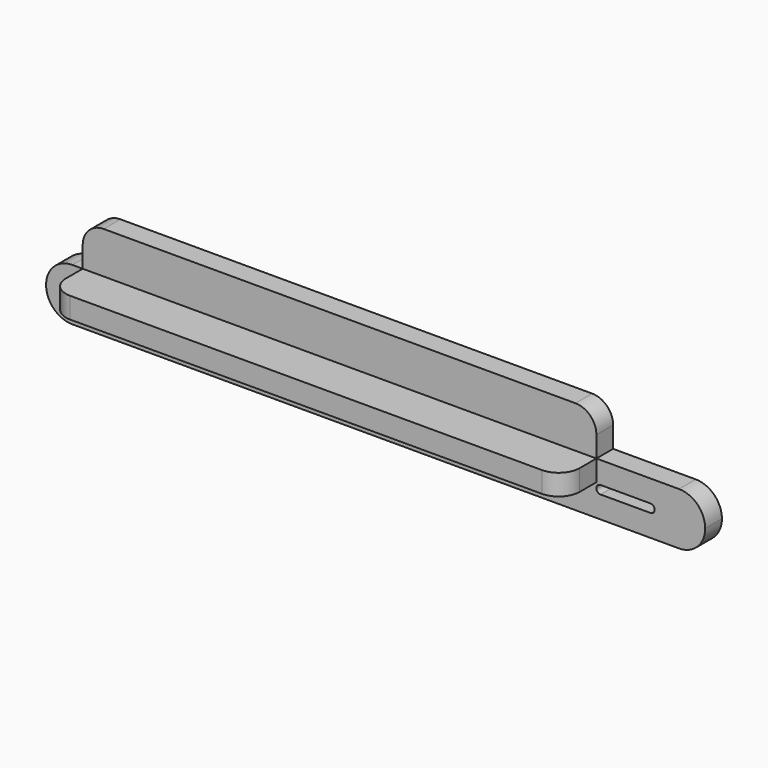
from build123d import *

# Parameters (mm, degrees)
F0_W     = 315
F0_H     = 25
F0_R     = 2.5
F1_DEPTH = 10
F2_R     = 12.49999
F3_W     = 245.5
F3_H     = 10
F4_DEPTH = 20
F5_W     = 245.5
F5_H     = 10
F6_DEPTH = 20
F7_R     = 10
F8_R     = 10


# Not quite as in the source:
# - a fillet or chamfer is up to 0.001 mm smaller than in the source, because OpenCascade refuses the exact size


with BuildPart() as f1:
    # F0 (on Front) → F1 (new body)
    with BuildSketch(Plane.XZ):
        with Locations((167.5, 12.5)):
            Rectangle(F0_W, F0_H)
        with Locations((25, 12.5)):
            Circle(F0_R, mode=Mode.SUBTRACT)
        with BuildLine():
            ThreePointArc((298.861, 14.5), (300.861, 12.5), (298.861, 10.5))
            Line((298.861, 10.5), (275, 10.5))
            ThreePointArc((275, 10.5), (273, 12.5), (275, 14.5))
            Line((275, 14.5), (298.861, 14.5))
        make_face(mode=Mode.SUBTRACT)
    extrude(amount=F1_DEPTH)

    # F2 (radius 12.5 in the source; OpenCascade refuses exactly that, so slightly less here)
    f2_edges = [f1.edges().sort_by_distance(p)[0] for p in [
        (10, -5, 25),
        (10, -5, 0),
        (325, -5, 0),
        (325, -5, 25),
    ]]
    fillet(f2_edges, radius=F2_R)

    # F3 (on face) → F4 (join)
    with BuildSketch(Plane.XZ.offset(10)):
        with Locations((150.25, 20)):
            Rectangle(F3_W, F3_H)
    extrude(amount=F4_DEPTH)

    # F5 (on face) → F6 (join)
    with BuildSketch(Plane.XY.offset(25)):
        with Locations((150.25, -5)):
            Rectangle(F5_W, F5_H)
    extrude(amount=F6_DEPTH)

    # F7
    f7_edges = [f1.edges().sort_by_distance(p)[0] for p in [
        (27.5, -5, 45),
    ]]
    fillet(f7_edges, radius=F7_R)

    # F8
    f8_edges = [f1.edges().sort_by_distance(p)[0] for p in [
        (273, -5, 45),
        (273, -30, 20),
        (27.5, -30, 20),
    ]]
    fillet(f8_edges, radius=F8_R)


solid = f1.part
